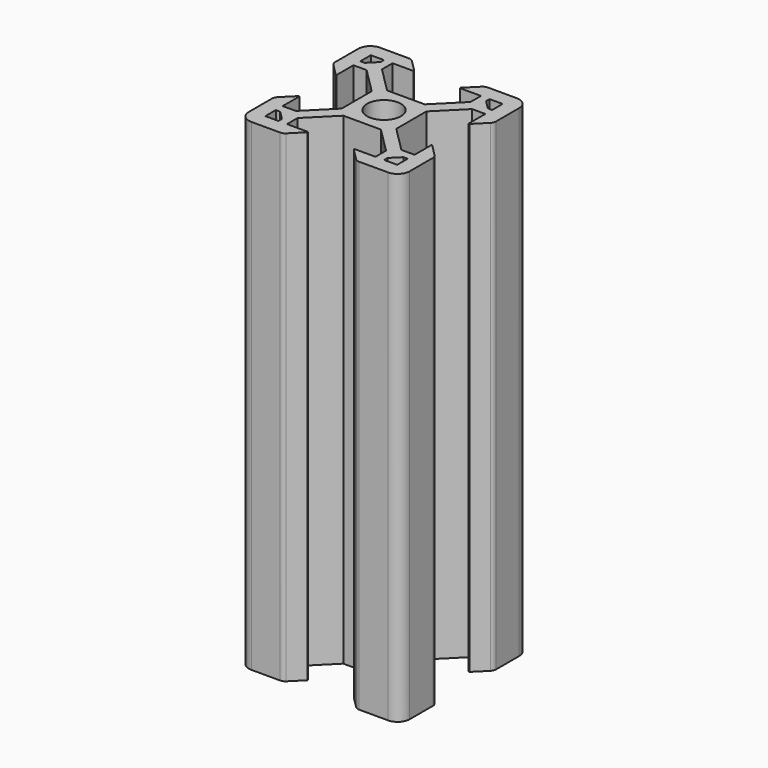
from build123d import *

# Parameters (mm, degrees)
F0_R     = 2.1
F1_DEPTH = 60


# Not quite as in the source:
# - ends of sketch curves that miss each other by under 0.0002 mm in the source are joined


with BuildPart() as f1:
    # F0 (on Top) → F1 (new body)
    with BuildSketch(Plane.XY):
        with BuildLine():
            Line((-8.2, 5.5), (-6.56066, 5.5))
            Line((-6.56066, 5.5), (-3.4, 2.33934))
            Line((-3.4, 2.33934), (-3.4, -2.33934))
            Line((-3.4, -2.33934), (-6.56066, -5.5))
            Line((-6.56066, -5.5), (-8.2, -5.5))
            Line((-8.2, -5.5), (-8.2, -2.89))
            Line((-8.2, -2.89), (-8.31, -2.89))
            Line((-8.31, -2.89), (-9.768614, -4.348614))
            ThreePointArc((-9.768614, -4.348614), (-9.9398646954, -4.6049087618), (-10, -4.907229))
            Line((-10, -4.907229), (-10, -8.5))
            ThreePointArc((-10, -8.5), (-9.5606601718, -9.5606601718), (-8.5, -10))
            Line((-8.5, -10), (-4.907229, -10))
            ThreePointArc((-4.907229, -10), (-4.6049087618, -9.9398646954), (-4.3486141429, -9.7686138571))
            Line((-4.3486141429, -9.7686138571), (-2.89, -8.31))
            Line((-2.89, -8.31), (-2.89, -8.2))
            Line((-2.89, -8.2), (-5.5, -8.2))
            Line((-5.5, -8.2), (-5.5, -6.56066))
            Line((-5.5, -6.56066), (-2.33934, -3.4))
            Line((-2.33934, -3.4), (2.33934, -3.4))
            Line((2.33934, -3.4), (5.5, -6.56066))
            Line((5.5, -6.56066), (5.5, -8.2))
            Line((5.5, -8.2), (2.89, -8.2))
            Line((2.89, -8.2), (2.89, -8.31))
            Line((2.89, -8.31), (4.348614, -9.768614))
            ThreePointArc((4.348614, -9.768614), (4.6049087618, -9.9398646954), (4.907229, -10))
            Line((4.907229, -10), (8.5, -10))
            ThreePointArc((8.5, -10), (9.5606601718, -9.5606601718), (10, -8.5))
            Line((10, -8.5), (10, -4.907229))
            ThreePointArc((10, -4.907229), (9.9398646954, -4.6049087618), (9.7686138571, -4.3486141429))
            Line((9.7686138571, -4.3486141429), (8.31, -2.89))
            Line((8.31, -2.89), (8.2, -2.89))
            Line((8.2, -2.89), (8.2, -5.5))
            Line((8.2, -5.5), (6.56066, -5.5))
            Line((6.56066, -5.5), (3.4, -2.33934))
            Line((3.4, -2.33934), (3.4, 2.33934))
            Line((3.4, 2.33934), (6.56066, 5.5))
            Line((6.56066, 5.5), (8.2, 5.5))
            Line((8.2, 5.5), (8.2, 2.89))
            Line((8.2, 2.89), (8.31, 2.89))
            Line((8.31, 2.89), (9.768614, 4.348614))
            ThreePointArc((9.768614, 4.348614), (9.9398646954, 4.6049087618), (10, 4.907229))
            Line((10, 4.907229), (10, 8.5))
            ThreePointArc((10, 8.5), (9.5606601718, 9.5606601718), (8.5, 10))
            Line((8.5, 10), (4.907229, 10))
            ThreePointArc((4.907229, 10), (4.6049087618, 9.9398646954), (4.3486141429, 9.7686138571))
            Line((4.3486141429, 9.7686138571), (2.89, 8.31))
            Line((2.89, 8.31), (2.89, 8.2))
            Line((2.89, 8.2), (5.5, 8.2))
            Line((5.5, 8.2), (5.5, 6.56066))
            Line((5.5, 6.56066), (2.33934, 3.4))
            Line((2.33934, 3.4), (-2.33934, 3.4))
            Line((-2.33934, 3.4), (-5.5, 6.56066))
            Line((-5.5, 6.56066), (-5.5, 8.2))
            Line((-5.5, 8.2), (-2.89, 8.2))
            Line((-2.89, 8.2), (-2.89, 8.31))
            Line((-2.89, 8.31), (-4.348614, 9.768614))
            ThreePointArc((-4.348614, 9.768614), (-4.6049087618, 9.9398646954), (-4.907229, 10))
            Line((-4.907229, 10), (-8.5, 10))
            ThreePointArc((-8.5, 10), (-9.5606601718, 9.5606601718), (-10, 8.5))
            Line((-10, 8.5), (-10, 4.907229))
            ThreePointArc((-10, 4.907229), (-9.9398646954, 4.6049087618), (-9.7686138571, 4.3486141429))
            Line((-9.7686138571, 4.3486141429), (-8.31, 2.89))
            Line((-8.31, 2.89), (-8.2, 2.89))
            Line((-8.2, 2.89), (-8.2, 5.5))
        make_face()
        Polygon((-6.57, -8.2), (-8.2, -8.2), (-8.2, -6.57), (-7.66, -6.57), (-6.57, -7.66), align=None, mode=Mode.SUBTRACT)
        Polygon((6.57, -7.66), (7.66, -6.57), (8.2, -6.57), (8.2, -8.2), (6.57, -8.2), align=None, mode=Mode.SUBTRACT)
        Polygon((-6.57, 7.66), (-7.66, 6.57), (-8.2, 6.57), (-8.2, 8.2), (-6.57, 8.2), align=None, mode=Mode.SUBTRACT)
        Circle(F0_R, mode=Mode.SUBTRACT)
        Polygon((6.57, 8.2), (8.2, 8.2), (8.2, 6.57), (7.66, 6.57), (6.57, 7.66), align=None, mode=Mode.SUBTRACT)
    extrude(amount=F1_DEPTH)


solid = f1.part
